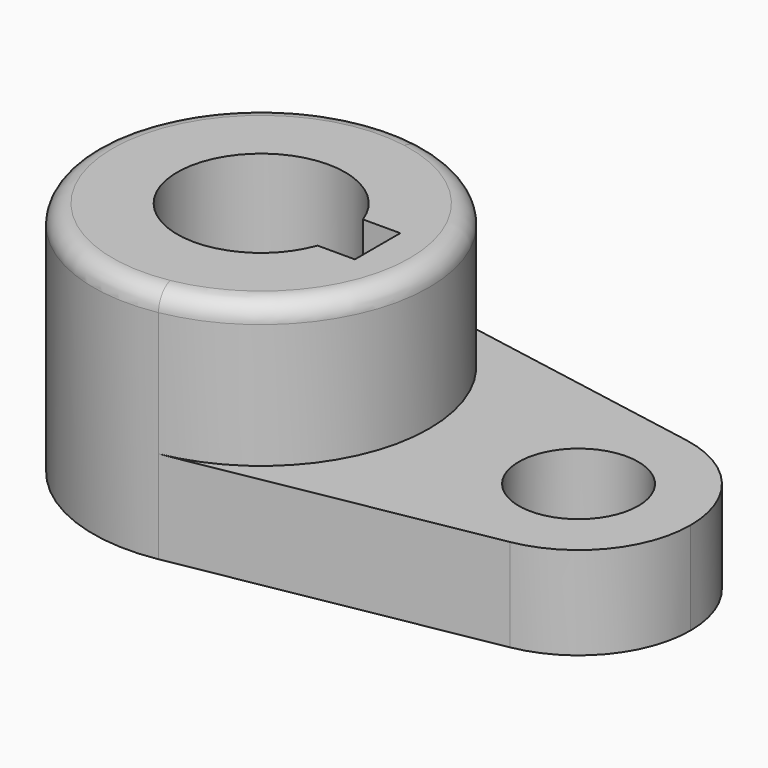
from build123d import *

# Parameters (mm, degrees)
F1_DEPTH = 40.2336
F0_R     = 10.16
F2_DEPTH = 15.7734
F3_R     = 3.302


# Not quite as in the source:
# - a feature names something its author has since deleted; it is built from what else it names


with BuildPart() as f1:
    # F0 (on Top) → F1 (new body)
    with BuildSketch(Plane.XY):
        with BuildLine():
            ThreePointArc((-48.9323529412, -28.1265414802), (-32.0589754437, -18.3362616868), (-25.4, 0))
            ThreePointArc((-25.4, 0), (-32.0589754437, 18.3362616868), (-48.9323529412, 28.1265414802))
            ThreePointArc((-48.9323529412, 28.1265414802), (-82.55, 0), (-48.9323529412, -28.1265414802))
        make_face()
        with BuildLine():
            ThreePointArc((-40.5272351207, -4.826), (-68.2625, 0), (-40.5272351207, 4.826))
            Line((-40.5272351207, 4.826), (-34.1772351207, 4.826))
            Line((-34.1772351207, 4.826), (-34.1772351207, -4.826))
            Line((-34.1772351207, -4.826), (-40.5272351207, -4.826))
        make_face(mode=Mode.SUBTRACT)
    extrude(amount=F1_DEPTH)

    # F0 (on Top) → F2 (join)
    with BuildSketch(Plane.XY):
        with BuildLine():
            ThreePointArc((-48.9323529412, 28.1265414802), (-32.0589754437, 18.3362616868), (-25.4, 0))
            ThreePointArc((-25.4, 0), (-32.0589754437, -18.3362616868), (-48.9323529412, -28.1265414802))
            Line((-48.9323529412, -28.1265414802), (3.3617647059, -18.7510276535))
            ThreePointArc((3.3617647059, -18.7510276535), (-19.05, 0), (3.3617647059, 18.7510276535))
            Line((3.3617647059, 18.7510276535), (-48.9323529412, 28.1265414802))
        make_face()
        with BuildLine():
            ThreePointArc((19.05, 0), (14.6106830375, 12.2241744579), (3.3617647059, 18.7510276535))
            ThreePointArc((3.3617647059, 18.7510276535), (-19.05, 0), (3.3617647059, -18.7510276535))
            ThreePointArc((3.3617647059, -18.7510276535), (14.6106830375, -12.2241744579), (19.05, 0))
        make_face()
        Circle(F0_R, mode=Mode.SUBTRACT)
    extrude(amount=F2_DEPTH)

    # F3
    f3_edges = [f1.edges().sort_by_distance(p)[0] for p in [
        (-59.017647, 28.126541, 40.2336),
    ]]
    fillet(f3_edges, radius=F3_R)


solid = f1.part
